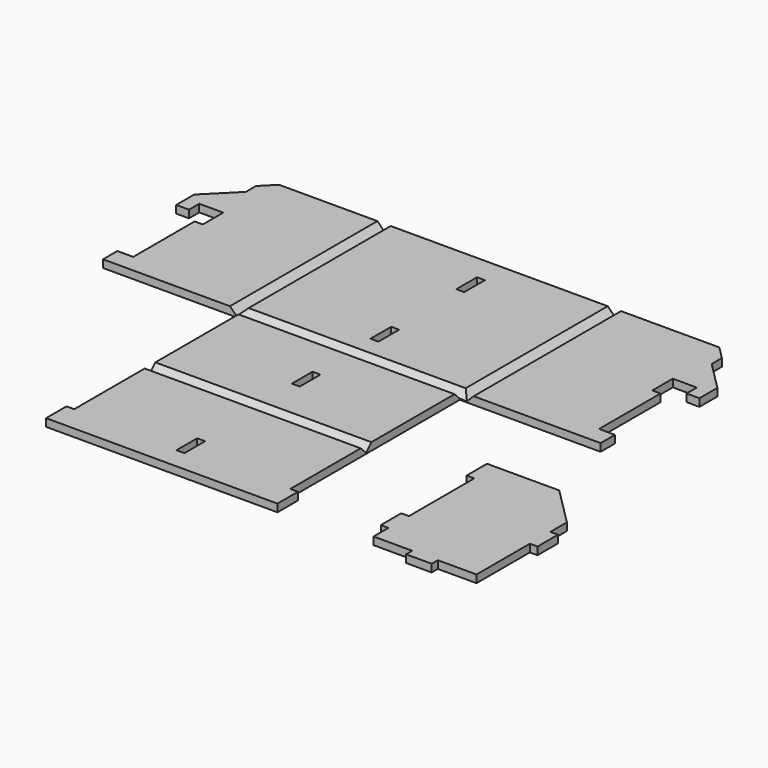
from build123d import *

# Parameters (mm, degrees)
F1_DEPTH   = 2.6
F2_SIZE    = 2.59999
F2_2_SIZE  = 2.59999
F3_DEPTH   = 2.6
F4_SIZE    = 2.59999
F5_W       = 3.1
F5_H       = 10.1
F6_DEPTH   = 4
F0_W       = 84.4
F0_H       = 45.8
F7_DEPTH   = 2.6
F8_SIZE    = 2.59999
F0_H_2     = 47
F9_DEPTH   = 2.6
F10_SIZE   = 2.59999
F11_W      = 10
F11_H      = 2.6
F12_DEPTH  = 3
F15_W      = 3.1
F15_H      = 10.1
F14_W      = 3.1
F14_H      = 10.1
F16_DEPTH  = 4
F18_DEPTH  = 3
F19_SIZE   = 5
F19_2_SIZE = 5
F20_SIZE   = 15
F21_DEPTH  = 0.4
F22_DEPTH  = 0.4
F23_DEPTH  = 25
F24_SIZE   = 4.99999


# Not quite as in the source:
# - a fillet or chamfer is up to 0.001 mm smaller than in the source, because OpenCascade refuses the exact size


with BuildPart() as f1:
    # F0 (on Top) → F1 (new body)
    with BuildSketch(Plane.XY):
        Polygon((-45, -36), (-45, 36), (-91, 36), (-91, 26), (-102.2, 14.8), (-102.2, 6), (-97.2, 6), (-97.2, 11), (-91, 11), (-87.8, 11), (-87.8, 1), (-91, 1), (-91, -29), (-97.2, -29), (-97.2, -36), (-91, -36), align=None)
    extrude(amount=F1_DEPTH)

    # F2#2 (size 2.6 in the source; OpenCascade refuses exactly that, so slightly less here)
    f2_2_edges = [f1.edges().sort_by_distance(p)[0] for p in [
        (-45, 0, 2.6),
    ]]
    chamfer(f2_2_edges, length=F2_2_SIZE)

    # F19#2
    f19_2_edges = [f1.edges().sort_by_distance(p)[0] for p in [
        (-91, 36, 1.3),
    ]]
    chamfer(f19_2_edges, length=F19_2_SIZE)



with BuildPart() as f1b:
    # F0 (on Top) → F1, piece 2 (new body)
    with BuildSketch(Plane.XY):
        Polygon((45, 36), (45, -36), (91, -36), (97.2, -36), (97.2, -29), (91, -29), (91, 1), (87.8, 1), (87.8, 11), (91, 11), (97.2, 11), (97.2, 6), (102.2, 6), (102.2, 14.8), (91, 26), (91, 36), align=None)
    extrude(amount=F1_DEPTH)

    # F2 (size 2.6 in the source; OpenCascade refuses exactly that, so slightly less here)
    f2_edges = [f1b.edges().sort_by_distance(p)[0] for p in [
        (45, 0, 2.6),
    ]]
    chamfer(f2_edges, length=F2_SIZE)

    # F19
    f19_edges = [f1b.edges().sort_by_distance(p)[0] for p in [
        (91, 36, 1.3),
    ]]
    chamfer(f19_edges, length=F19_SIZE)


with BuildPart() as f3:
    # F0 (on Top) → F3 (new body)
    with BuildSketch(Plane.XY):
        Polygon((42.2, -36), (45, -36), (45, 36), (-45, 36), (-45, -36), (-42.2, -36), align=None)
    extrude(amount=F3_DEPTH)

    # F4 (size 2.6 in the source; OpenCascade refuses exactly that, so slightly less here)
    f4_edges = [f3.edges().sort_by_distance(p)[0] for p in [
        (45, 0, 2.6),
        (-45, 0, 2.6),
        (0, -36, 2.6),
    ]]
    chamfer(f4_edges, length=F4_SIZE)

    # F5 (on face) → F6 (cut)
    with BuildSketch(Plane.XY.offset(2.6)):
        with Locations((0.85, 20.95)):
            Rectangle(F5_W, F5_H)
        with Locations((0.85, -20.95)):
            Rectangle(F5_W, F5_H)
    extrude(amount=-F6_DEPTH, mode=Mode.SUBTRACT)


with BuildPart() as f7:
    # F0 (on Top) → F7 (new body)
    with BuildSketch(Plane.XY):
        with Locations((0, -58.9)):
            Rectangle(F0_W, F0_H)
    extrude(amount=F7_DEPTH)

    # F8 (size 2.6 in the source; OpenCascade refuses exactly that, so slightly less here)
    f8_edges = [f7.edges().sort_by_distance(p)[0] for p in [
        (0, -36, 2.6),
        (0, -81.8, 2.6),
    ]]
    chamfer(f8_edges, length=F8_SIZE)


with BuildPart() as f9:
    # F0 (on Top) → F9 (new body)
    with BuildSketch(Plane.XY):
        with Locations((0, -105.3)):
            Rectangle(F0_W, F0_H_2)
    extrude(amount=F9_DEPTH)

    # F10 (size 2.6 in the source; OpenCascade refuses exactly that, so slightly less here)
    f10_edges = [f9.edges().sort_by_distance(p)[0] for p in [
        (0, -81.8, 2.6),
    ]]
    chamfer(f10_edges, length=F10_SIZE)

    # F13: F12 across plane


with BuildPart() as f12:
    # F11 (on face) → F12 (new body)
    with BuildSketch(Plane(origin=(-42.2, 0, 0), x_dir=(0, -1, 0), z_dir=(-1, 0, 0))):
        with Locations((123.8, 1.3)):
            Rectangle(F11_W, F11_H)
    extrude(amount=F12_DEPTH)


with BuildPart() as f9_1:
    add(f9.part)
    add(f12.part.mirror(Plane.YZ))


with BuildPart() as f16_tool:
    # F15 (on face) + F14 (on face) → F16 (new body)
    with BuildSketch(Plane.XY.offset(2.6)):
        with Locations((0.65, -115.45)):
            Rectangle(F15_W, F15_H)
    with BuildSketch(Plane.XY.offset(2.6)):
        with Locations((0.65, -59.1)):
            Rectangle(F14_W, F14_H)
    extrude(amount=-F16_DEPTH)


with BuildPart() as f7_1:
    add(f7.part)

    # F16: cut by f16_tool
    add(f16_tool.part, mode=Mode.SUBTRACT)


with BuildPart() as f9_2:
    add(f9_1.part)

    # F16: cut by f16_tool
    add(f16_tool.part, mode=Mode.SUBTRACT)


with BuildPart() as f18:
    # F17 (on Top) → F18 (new body)
    with BuildSketch(Plane.XY):
        Polygon((122.3451334953, -68.8853332162), (82.1451334953, -68.8853332162), (79.1451334953, -68.8853332162), (79.1451334953, -78.8853332162), (82.1451334953, -78.8853332162), (82.1451334953, -110.7853332162), (79.1451334953, -110.7853332162), (79.1451334953, -120.7853332162), (82.1451334953, -120.7853332162), (82.1451334953, -128.0353332162), (97.2451334953, -128.0353332162), (97.2451334953, -131.0353332162), (102.2451334953, -131.0353332162), (107.2451334953, -131.0353332162), (107.2451334953, -128.0353332162), (122.3451334953, -128.0353332162), (122.3451334953, -101.9853332162), (125.3451334953, -101.9853332162), (125.3451334953, -91.9853332162), (122.3451334953, -91.9853332162), align=None)
    extrude(amount=F18_DEPTH)

    # F20
    f20_edges = [f18.edges().sort_by_distance(p)[0] for p in [
        (122.345133, -68.885333, 1.5),
    ]]
    chamfer(f20_edges, length=F20_SIZE)


with BuildPart() as f1_1:
    add(f1.part)

    add(f1b.part)  # F21 merges F1b

    add(f3.part)  # F21 merges F3

    add(f7_1.part)  # F21 merges F7

    add(f9_2.part)  # F21 merges F9

    add(f12.part)  # F21 merges F12
    # F0 (on Top) → F21 (join)
    with BuildSketch(Plane.XY):
        Polygon((45, 36), (45, -36), (91, -36), (97.2, -36), (97.2, -29), (91, -29), (91, 1), (87.8, 1), (87.8, 11), (91, 11), (97.2, 11), (97.2, 6), (102.2, 6), (102.2, 14.8), (91, 26), (91, 36), align=None)
        Polygon((-45, -36), (-45, 36), (-91, 36), (-91, 26), (-102.2, 14.8), (-102.2, 6), (-97.2, 6), (-97.2, 11), (-91, 11), (-87.8, 11), (-87.8, 1), (-91, 1), (-91, -29), (-97.2, -29), (-97.2, -36), (-91, -36), align=None)
        with Locations((0, -105.3)):
            Rectangle(F0_W, F0_H_2)
        with Locations((0, -58.9)):
            Rectangle(F0_W, F0_H)
        Polygon((42.2, -36), (45, -36), (45, 36), (-45, 36), (-45, -36), (-42.2, -36), align=None)
    extrude(amount=-F21_DEPTH)

    # F22 (add): faces of the model
    f22_faces = [f1_1.faces().sort_by_distance(p)[0] for p in [
        (43.7, -123.8, 0),
        (-43.7, -123.8, 0),
    ]]
    extrude(f22_faces, amount=F22_DEPTH)

    # F15 (on face) + F14 (on face) + F5 (on face) → F23 (cut)
    with BuildSketch(Plane.XY.offset(2.6)):
        with Locations((0.65, -115.45)):
            Rectangle(F15_W, F15_H)
    with BuildSketch(Plane.XY.offset(2.6)):
        with Locations((0.65, -59.1)):
            Rectangle(F14_W, F14_H)
    with BuildSketch(Plane.XY.offset(2.6)):
        with Locations((0.85, 20.95)):
            Rectangle(F5_W, F5_H)
        with Locations((0.85, -20.95)):
            Rectangle(F5_W, F5_H)
    extrude(amount=-F23_DEPTH, mode=Mode.SUBTRACT)

    # F24 (size 5 in the source; OpenCascade refuses exactly that, so slightly less here)
    f24_edges = [f1_1.edges().sort_by_distance(p)[0] for p in [
        (-91, 36, -0.2),
        (91, 36, -0.2),
    ]]
    chamfer(f24_edges, length=F24_SIZE)


solid = Compound([f18.part, f1_1.part])
